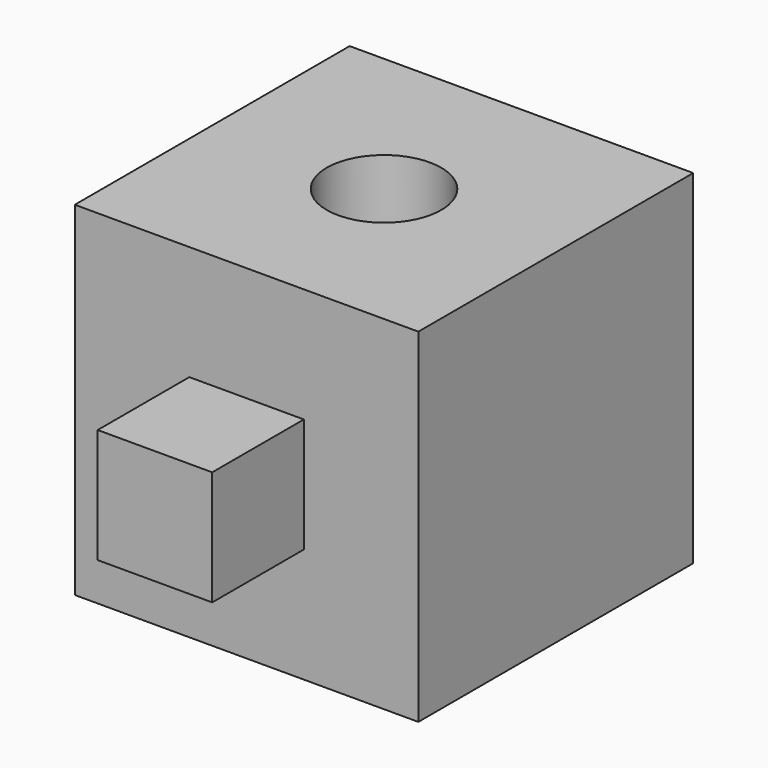
from build123d import *

# Parameters (mm, degrees)
F0_W     = 76.2
F0_H     = 76.2
F1_DEPTH = 76.2
F2_W     = 25.4
F2_H     = 25.4
F3_DEPTH = 25.4
F5_D     = 25.4


# Not quite as in the source:
# - the program builds the solid bodies; features that only make, move or delete a surface that nothing else refers to are left out


with BuildPart() as f1:
    # F0 (on Front) → F1 (new body)
    with BuildSketch(Plane.XZ):
        with Locations((38.1, 38.1)):
            Rectangle(F0_W, F0_H)
    extrude(amount=F1_DEPTH)

    # F2 (on face) → F3 (join)
    with BuildSketch(Plane.XZ.offset(76.2)):
        with Locations((38.1, 38.1)):
            Rectangle(F2_W, F2_H)
    extrude(amount=F3_DEPTH)

    # F5 (through all)
    with Locations(Plane.XY.offset(76.2)):
        with Locations((38.1, -38.1)):
            Hole(F5_D / 2)


solid = f1.part
